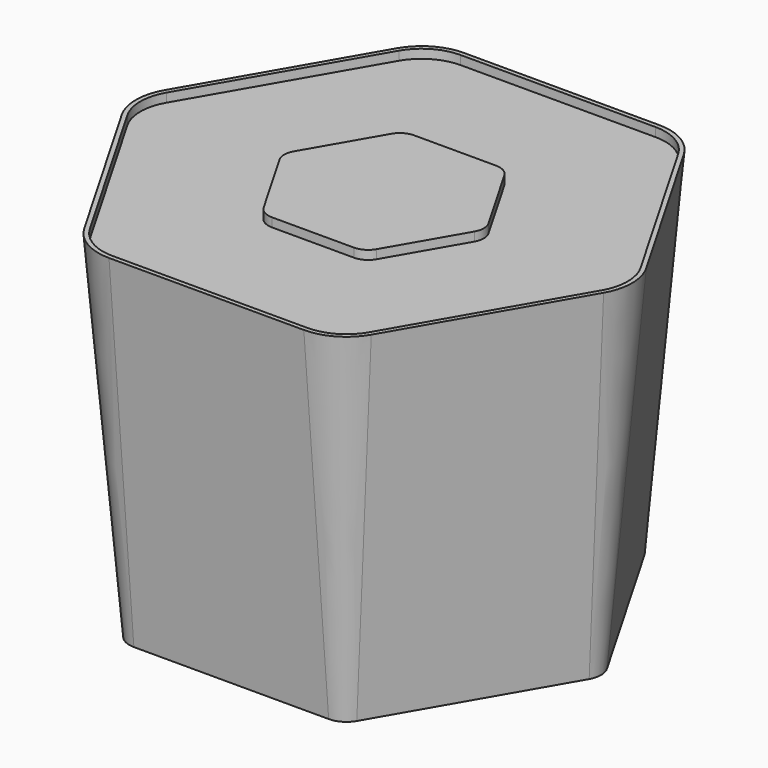
from build123d import *

# Parameters (mm, degrees)
F1_DEPTH = 400
F1_TAPER = 5
F2_DEPTH = 10


with BuildPart() as f1:
    # F0 (on Top) → F1 (new body)
    with BuildSketch(Plane.XY):
        with BuildLine():
            Line((109.696551146, 250), (-109.696551146, 250))
            ThreePointArc((-109.696551146, 250), (-139.696551146, 241.9615242271), (-161.6580753731, 220))
            Line((-161.6580753731, 220), (-271.3546265191, 30))
            ThreePointArc((-271.3546265191, 30), (-279.3931022921, 0), (-271.3546265191, -30))
            Line((-271.3546265191, -30), (-161.6580753731, -220))
            ThreePointArc((-161.6580753731, -220), (-139.696551146, -241.9615242271), (-109.696551146, -250))
            Line((-109.696551146, -250), (109.696551146, -250))
            ThreePointArc((109.696551146, -250), (139.696551146, -241.9615242271), (161.6580753731, -220))
            Line((161.6580753731, -220), (271.3546265191, -30))
            ThreePointArc((271.3546265191, -30), (279.3931022921, 0), (271.3546265191, 30))
            Line((271.3546265191, 30), (161.6580753731, 220))
            ThreePointArc((161.6580753731, 220), (139.696551146, 241.9615242271), (109.696551146, 250))
        make_face()
        with BuildLine():
            ThreePointArc((-109.696551146, -244.9999966036), (-137.1965494478, -237.6313942668), (-157.3279454128, -217.4999983018))
            Line((-157.3279454128, -217.4999983018), (-267.0244965589, -27.4999983018))
            ThreePointArc((-267.0244965589, -27.4999983018), (-274.3930988957, 0), (-267.0244965589, 27.4999983018))
            Line((-267.0244965589, 27.4999983018), (-157.3279454128, 217.4999983018))
            ThreePointArc((-157.3279454128, 217.4999983018), (-137.1965494478, 237.6313942668), (-109.696551146, 244.9999966036))
            Line((-109.696551146, 244.9999966036), (109.696551146, 244.9999966036))
            ThreePointArc((109.696551146, 244.9999966036), (137.1965494478, 237.6313942668), (157.3279454128, 217.4999983018))
            Line((157.3279454128, 217.4999983018), (267.0244965589, 27.4999983018))
            ThreePointArc((267.0244965589, 27.4999983018), (274.3930988957, 0), (267.0244965589, -27.4999983018))
            Line((267.0244965589, -27.4999983018), (157.3279454128, -217.4999983018))
            ThreePointArc((157.3279454128, -217.4999983018), (137.1965494478, -237.6313942668), (109.696551146, -244.9999966036))
            Line((109.696551146, -244.9999966036), (-109.696551146, -244.9999966036))
        make_face(mode=Mode.SUBTRACT)
        with BuildLine():
            Line((-267.0244965589, -27.4999983018), (-157.3279454128, -217.4999983018))
            ThreePointArc((-157.3279454128, -217.4999983018), (-137.1965494478, -237.6313942668), (-109.696551146, -244.9999966036))
            Line((-109.696551146, -244.9999966036), (109.696551146, -244.9999966036))
            ThreePointArc((109.696551146, -244.9999966036), (137.1965494478, -237.6313942668), (157.3279454128, -217.4999983018))
            Line((157.3279454128, -217.4999983018), (267.0244965589, -27.4999983018))
            ThreePointArc((267.0244965589, -27.4999983018), (274.3930988957, 0), (267.0244965589, 27.4999983018))
            Line((267.0244965589, 27.4999983018), (157.3279454128, 217.4999983018))
            ThreePointArc((157.3279454128, 217.4999983018), (137.1965494478, 237.6313942668), (109.696551146, 244.9999966036))
            Line((109.696551146, 244.9999966036), (-109.696551146, 244.9999966036))
            ThreePointArc((-109.696551146, 244.9999966036), (-137.1965494478, 237.6313942668), (-157.3279454128, 217.4999983018))
            Line((-157.3279454128, 217.4999983018), (-267.0244965589, 27.4999983018))
            ThreePointArc((-267.0244965589, 27.4999983018), (-274.3930988957, 0), (-267.0244965589, -27.4999983018))
        make_face()
        with BuildLine():
            ThreePointArc((-63.5085296109, 90), (-56.1880215352, 97.3205080757), (-46.1880215352, 100))
            Line((-46.1880215352, 100), (46.1880215352, 100))
            ThreePointArc((46.1880215352, 100), (56.1880215352, 97.3205080757), (63.5085296109, 90))
            Line((63.5085296109, 90), (109.696551146, 10))
            ThreePointArc((109.696551146, 10), (112.3760430703, 0), (109.696551146, -10))
            Line((109.696551146, -10), (63.5085296109, -90))
            ThreePointArc((63.5085296109, -90), (56.1880215352, -97.3205080757), (46.1880215352, -100))
            Line((46.1880215352, -100), (-46.1880215352, -100))
            ThreePointArc((-46.1880215352, -100), (-56.1880215352, -97.3205080757), (-63.5085296109, -90))
            Line((-63.5085296109, -90), (-109.696551146, -10))
            ThreePointArc((-109.696551146, -10), (-112.3760430703, 0), (-109.696551146, 10))
            Line((-109.696551146, 10), (-63.5085296109, 90))
        make_face(mode=Mode.SUBTRACT)
        with BuildLine():
            Line((46.1880215352, 100), (-46.1880215352, 100))
            ThreePointArc((-46.1880215352, 100), (-56.1880215352, 97.3205080757), (-63.5085296109, 90))
            Line((-63.5085296109, 90), (-109.696551146, 10))
            ThreePointArc((-109.696551146, 10), (-112.3760430703, 0), (-109.696551146, -10))
            Line((-109.696551146, -10), (-63.5085296109, -90))
            ThreePointArc((-63.5085296109, -90), (-56.1880215352, -97.3205080757), (-46.1880215352, -100))
            Line((-46.1880215352, -100), (46.1880215352, -100))
            ThreePointArc((46.1880215352, -100), (56.1880215352, -97.3205080757), (63.5085296109, -90))
            Line((63.5085296109, -90), (109.696551146, -10))
            ThreePointArc((109.696551146, -10), (112.3760430703, 0), (109.696551146, 10))
            Line((109.696551146, 10), (63.5085296109, 90))
            ThreePointArc((63.5085296109, 90), (56.1880215352, 97.3205080757), (46.1880215352, 100))
        make_face()
    extrude(amount=-F1_DEPTH, taper=F1_TAPER)

    # F0 (on Top) → F2 (cut)
    with BuildSketch(Plane.XY):
        with BuildLine():
            Line((-267.0244965589, -27.4999983018), (-157.3279454128, -217.4999983018))
            ThreePointArc((-157.3279454128, -217.4999983018), (-137.1965494478, -237.6313942668), (-109.696551146, -244.9999966036))
            Line((-109.696551146, -244.9999966036), (109.696551146, -244.9999966036))
            ThreePointArc((109.696551146, -244.9999966036), (137.1965494478, -237.6313942668), (157.3279454128, -217.4999983018))
            Line((157.3279454128, -217.4999983018), (267.0244965589, -27.4999983018))
            ThreePointArc((267.0244965589, -27.4999983018), (274.3930988957, 0), (267.0244965589, 27.4999983018))
            Line((267.0244965589, 27.4999983018), (157.3279454128, 217.4999983018))
            ThreePointArc((157.3279454128, 217.4999983018), (137.1965494478, 237.6313942668), (109.696551146, 244.9999966036))
            Line((109.696551146, 244.9999966036), (-109.696551146, 244.9999966036))
            ThreePointArc((-109.696551146, 244.9999966036), (-137.1965494478, 237.6313942668), (-157.3279454128, 217.4999983018))
            Line((-157.3279454128, 217.4999983018), (-267.0244965589, 27.4999983018))
            ThreePointArc((-267.0244965589, 27.4999983018), (-274.3930988957, 0), (-267.0244965589, -27.4999983018))
        make_face()
        with BuildLine():
            ThreePointArc((-63.5085296109, 90), (-56.1880215352, 97.3205080757), (-46.1880215352, 100))
            Line((-46.1880215352, 100), (46.1880215352, 100))
            ThreePointArc((46.1880215352, 100), (56.1880215352, 97.3205080757), (63.5085296109, 90))
            Line((63.5085296109, 90), (109.696551146, 10))
            ThreePointArc((109.696551146, 10), (112.3760430703, 0), (109.696551146, -10))
            Line((109.696551146, -10), (63.5085296109, -90))
            ThreePointArc((63.5085296109, -90), (56.1880215352, -97.3205080757), (46.1880215352, -100))
            Line((46.1880215352, -100), (-46.1880215352, -100))
            ThreePointArc((-46.1880215352, -100), (-56.1880215352, -97.3205080757), (-63.5085296109, -90))
            Line((-63.5085296109, -90), (-109.696551146, -10))
            ThreePointArc((-109.696551146, -10), (-112.3760430703, 0), (-109.696551146, 10))
            Line((-109.696551146, 10), (-63.5085296109, 90))
        make_face(mode=Mode.SUBTRACT)
    extrude(amount=-F2_DEPTH, mode=Mode.SUBTRACT)


solid = f1.part
